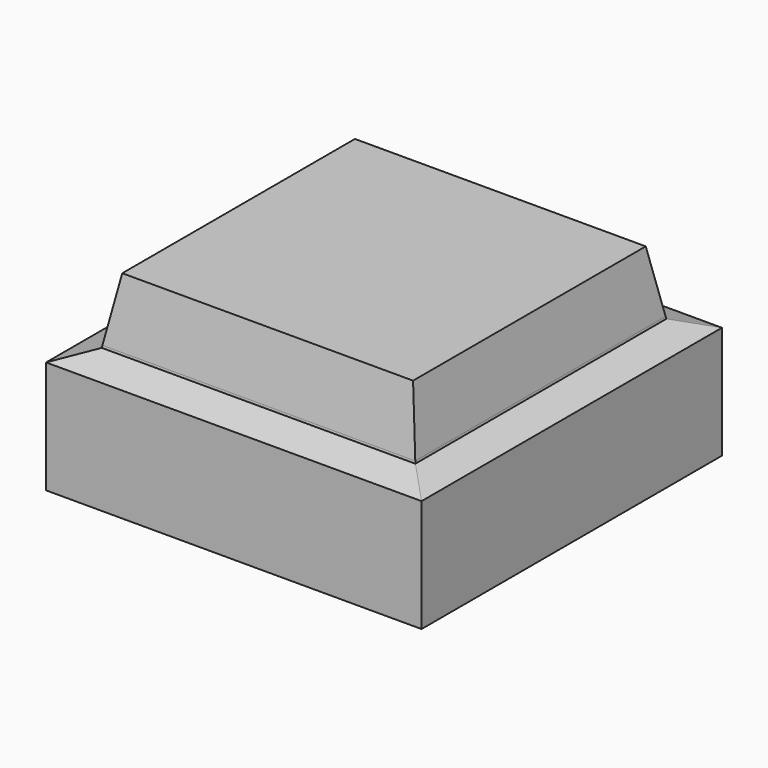
from build123d import *

# Parameters (mm, degrees)
F0_W          = 30
F0_H          = 30
F1_DEPTH      = 10
F2_T          = -2.5
F3_SIZE2      = 7.49999
F3_SIZE       = 0.99999
F4_W          = 25
F4_H          = 25
F5_DEPTH      = 5
F5_TAPER      = 10
F6_T          = 2.5
F6_T3_DEPTH   = 12.6321563139
F6_T5_DEPTH   = 12.6321563139
F6_T7_DEPTH   = 12.6321563139
F6_T9_DEPTH   = 12.6321563139
F6_T11_DEPTH  = 5.00001
F6_T13_DEPTH  = 30
F6_T15_DEPTH  = 30
F7_T4_DEPTH   = 45.5703660639
F7_T10_DEPTH  = 45.5703660639
F7_T16_DEPTH  = 45.5703660639
F7_T23_DEPTH  = 45.5703660639
F7_T29_DEPTH  = 45.5703660639
F7_T35_DEPTH  = 45.5703660639
F7_T41_DEPTH  = 45.5703660639
F7_T47_DEPTH  = 45.5703660639
F7_T54_DEPTH  = 45.5703660639
F7_T60_DEPTH  = 45.5703660639
F7_T66_DEPTH  = 45.5703660639
F7_T72_DEPTH  = 45.5703660639
F7_T78_DEPTH  = 45.5703660639
F7_T85_DEPTH  = 45.5703660639
F7_T91_DEPTH  = 45.5703660639
F7_T97_DEPTH  = 45.5703660639
F7_T103_DEPTH = 45.5703660639
F7_T109_DEPTH = 45.5703660639
F7_T116_DEPTH = 45.5703660639
F7_T122_DEPTH = 45.5703660639
F8_C1_SIZE2   = 1
F8_C1_SIZE    = 1.5
F8_C2_SIZE2   = 1
F8_C2_SIZE    = 1.5
F8_C3_SIZE2   = 1
F8_C3_SIZE    = 1.5
F8_C4_SIZE2   = 1
F8_C4_SIZE    = 1.5


# Not quite as in the source:
# - a fillet or chamfer that OpenCascade refuses, or shapes differently, is made with other operations: its cross-section is extruded or revolved along the edge and cut away or added
# - a fillet or chamfer is up to 0.001 mm smaller than in the source, because OpenCascade refuses the exact size
# - a shell that OpenCascade refuses in one call is made with other operations: the cavity is built on its own and cut out


with BuildPart() as f1:
    # F0 (on Top) → F1 (new body)
    with BuildSketch(Plane.XY):
        with Locations((15, 15)):
            Rectangle(F0_W, F0_H)
    extrude(amount=F1_DEPTH)

    # F2
    f2_openings = [f1.faces().sort_by_distance(p)[0] for p in [
        (15, 15, 0),
    ]]
    offset(amount=F2_T, openings=f2_openings)

    # F3 (size 1 and 7.5 in the source; OpenCascade refuses exactly that, so slightly less here)
    f3_edges = [f1.edges().sort_by_distance(p)[0] for p in [
        (27.5, 15, 0),
        (15, 27.5, 0),
        (2.5, 15, 0),
        (15, 2.5, 0),
    ]]
    chamfer(f3_edges, length=F3_SIZE, length2=F3_SIZE2)

    # F4 (on face) → F5 (join)
    with BuildSketch(Plane.XY.offset(10)):
        with Locations((15, 15)):
            Rectangle(F4_W, F4_H)
    extrude(amount=F5_DEPTH, taper=F5_TAPER)

    # F6: shell of thickness 2.5, made by hand


with BuildPart() as f6_core1:
    # F6_t2: copy of F1
    add(f1.part)

    # the walls: a layer under each face that stays
    f6_faces = [f6_core1.faces().sort_by_distance(p)[0] for p in [
        (1, 1, 0),
        (27.999995, 15, 3.749995),
        (15, 2.000005, 3.749995),
        (15, 27.999995, 3.749995),
        (2.000005, 15, 3.749995),
        (0, 15, 5),
        (15, 0, 5),
        (30, 15, 5),
        (15, 30, 5),
        (27.5, 15, 7.499995),
        (15, 2.5, 7.499995),
        (15, 27.5, 7.499995),
        (2.5, 15, 7.499995),
        (2.1428571429, 2.1428571429, 10),
        (27.0591825482, 15, 12.5),
        (15, 27.0591825482, 12.5),
        (2.9408174518, 15, 12.5),
        (15, 2.9408174518, 12.5),
        (15, 15, 15),
    ]]
    thicken(f6_faces, amount=-F6_T, mode=Mode.SUBTRACT)

    # F6_s4 → F6_t3 (cut)
    with BuildSketch(Plane(origin=(0.7910693611, -0.7910693611, -5.9330716286), x_dir=(-0.7071067812, -0.7071067812, 0), z_dir=(-0.1310232599, 0.1310232599, 0.9826829655))):
        Polygon((-21.2132034356, 18.7255916199), (-22.9654636265, 20.5443932655), (-21.2132034356, 22.2663095063), (-19.4609432447, 20.5443932655), align=None)
    extrude(amount=F6_T3_DEPTH, mode=Mode.SUBTRACT)

    # F6_s6 → F6_t5 (cut)
    with BuildSketch(Plane(origin=(1.3060821999, 1.3060821999, -9.7957013952), x_dir=(0.7071067812, -0.7071067812, 0), z_dir=(-0.1310232599, -0.1310232599, 0.9826829655))):
        Polygon((0, 39.5714452805), (1.7522601909, 41.3902469261), (0, 43.1121631669), (-1.7522601909, 41.3902469261), align=None)
    extrude(amount=F6_T5_DEPTH, mode=Mode.SUBTRACT)

    # F6_s8 → F6_t7 (cut)
    with BuildSketch(Plane(origin=(-0.2760565224, -0.2760565224, -2.0704418621), x_dir=(-0.7071067812, 0.7071067812, 0), z_dir=(0.1310232599, 0.1310232599, 0.9826829655))):
        Polygon((0, -2.1202620407), (-1.7522601909, -0.3014603951), (0, 1.4204558457), (1.7522601909, -0.3014603951), align=None)
    extrude(amount=F6_T7_DEPTH, mode=Mode.SUBTRACT)

    # F6_s10 → F6_t9 (cut)
    with BuildSketch(Plane(origin=(-0.7910693611, 0.7910693611, -5.9330716286), x_dir=(0.7071067812, 0.7071067812, 0), z_dir=(0.1310232599, -0.1310232599, 0.9826829655))):
        Polygon((21.2132034356, 18.7255916199), (22.9654636265, 20.5443932655), (21.2132034356, 22.2663095063), (19.4609432447, 20.5443932655), align=None)
    extrude(amount=F6_T9_DEPTH, mode=Mode.SUBTRACT)

    # F6_s12 → F6_t11 (cut)
    with BuildSketch(Plane.XY.offset(4.99999)):
        Polygon((27.475, 2.525), (30, 2.5), (30, 0), (27.5, 0), align=None)
        Polygon((27.475, 27.475), (30, 27.5), (30, 30), (27.5, 30), align=None)
        Polygon((2.525, 2.525), (2.5, 0), (0, 0), (0, 2.5), align=None)
        Polygon((2.525, 27.475), (2.5, 30), (0, 30), (0, 27.5), align=None)
    extrude(amount=F6_T11_DEPTH, mode=Mode.SUBTRACT)

    # F6_s14 → F6_t13 (cut)
    with BuildSketch(Plane.XZ.offset(-30)):
        Polygon((27.5246201938, 10.0293412044), (27.5, 7.5), (25.4022509221, 7.5), (25.0379806175, 9.5658795558), align=None)
        Polygon((2.4753798062, 10.0293412044), (2.5, 7.5), (4.5977490779, 7.5), (4.9620193825, 9.5658795558), align=None)
    extrude(amount=F6_T13_DEPTH, mode=Mode.SUBTRACT)

    # F6_s16 → F6_t15 (cut)
    with BuildSketch(Plane.YZ):
        Polygon((27.5246201938, 10.0293412044), (27.5, 7.5), (25.4022509221, 7.5), (25.0379806175, 9.5658795558), align=None)
        Polygon((2.4753798062, 10.0293412044), (2.5, 7.5), (4.5977490779, 7.5), (4.9620193825, 9.5658795558), align=None)
    extrude(amount=F6_T15_DEPTH, mode=Mode.SUBTRACT)


with BuildPart() as f1_1:
    add(f1.part)

    # what is left inside the walls is the cavity
    f6_cavity = [f6_core1.part.solids().sort_by_distance(p)[0] for p in [
        (15, 11.532583, 7.525),
    ]]
    add(f6_cavity, mode=Mode.SUBTRACT)

    # F7: chamfer of 1 x 3 on 4 edges, made by hand


with BuildPart() as f7_tool2:
    # F7_s3 → F7_t4 (new body)
    with BuildSketch(Plane.XZ.offset(7.785183032)):
        Polygon((30, 9), (27, 10), (30, 10), align=None)
    extrude(amount=-F7_T4_DEPTH)

    split(bisect_by=Plane(origin=(28.3808742524, 0, 5.0043138668), x_dir=(0, 1, 0), z_dir=(0.984807753, 0, 0.1736481777)), keep=Keep.TOP)

    split(bisect_by=Plane(origin=(0, 0.7145150594, -0.1259882831), x_dir=(1, 0, 0), z_dir=(0, -0.984807753, 0.1736481777)), keep=Keep.TOP)


with BuildPart() as f1_2:
    add(f1_1.part)

    # F7_t1: cut F7_tool2
    add(f7_tool2.part, mode=Mode.SUBTRACT)


with BuildPart() as f7_tool8:
    # F7_s9 → F7_t10 (new body)
    with BuildSketch(Plane.XZ.offset(7.785183032)):
        Polygon((30, 9), (27, 10), (30, 10), align=None)
    extrude(amount=-F7_T10_DEPTH)

    split(bisect_by=Plane(origin=(28.3808742524, 0, 5.0043138668), x_dir=(0, 1, 0), z_dir=(-0.984807753, 0, -0.1736481777)), keep=Keep.TOP)

    split(bisect_by=Plane(origin=(0, 0.7145150594, -0.1259882831), x_dir=(1, 0, 0), z_dir=(0, -0.984807753, 0.1736481777)), keep=Keep.TOP)


with BuildPart() as f1_3:
    add(f1_2.part)

    # F7_t7: cut F7_tool8
    add(f7_tool8.part, mode=Mode.SUBTRACT)


with BuildPart() as f7_tool14:
    # F7_s15 → F7_t16 (new body)
    with BuildSketch(Plane.XZ.offset(7.785183032)):
        Polygon((30, 9), (27, 10), (30, 10), align=None)
    extrude(amount=-F7_T16_DEPTH)

    split(bisect_by=Plane(origin=(28.3808742524, 0, 5.0043138668), x_dir=(0, 1, 0), z_dir=(0.984807753, 0, 0.1736481777)), keep=Keep.TOP)

    split(bisect_by=Plane(origin=(0, 28.3808742524, 5.0043138668), x_dir=(1, 0, 0), z_dir=(0, -0.984807753, -0.1736481777)), keep=Keep.TOP)

    split(bisect_by=Plane(origin=(0, 0.7145150594, -0.1259882831), x_dir=(1, 0, 0), z_dir=(0, 0.984807753, -0.1736481777)), keep=Keep.TOP)


with BuildPart() as f1_4:
    add(f1_3.part)

    # F7_t13: cut F7_tool14
    add(f7_tool14.part, mode=Mode.SUBTRACT)


with BuildPart() as f7_tool21:
    # F7_s22 → F7_t23 (new body)
    with BuildSketch(Plane.XZ.offset(7.785183032)):
        Polygon((30, 9), (27, 10), (30, 10), align=None)
    extrude(amount=-F7_T23_DEPTH)

    split(bisect_by=Plane(origin=(28.3808742524, 0, 5.0043138668), x_dir=(0, 1, 0), z_dir=(0.984807753, 0, 0.1736481777)), keep=Keep.TOP)

    split(bisect_by=Plane(origin=(0, 28.3808742524, 5.0043138668), x_dir=(1, 0, 0), z_dir=(0, 0.984807753, 0.1736481777)), keep=Keep.TOP)


with BuildPart() as f1_5:
    add(f1_4.part)

    # F7_t20: cut F7_tool21
    add(f7_tool21.part, mode=Mode.SUBTRACT)


with BuildPart() as f7_tool27:
    # F7_s28 → F7_t29 (new body)
    with BuildSketch(Plane.XZ.offset(7.785183032)):
        Polygon((30, 9), (27, 10), (30, 10), align=None)
    extrude(amount=-F7_T29_DEPTH)

    split(bisect_by=Plane(origin=(28.3808742524, 0, 5.0043138668), x_dir=(0, 1, 0), z_dir=(-0.984807753, 0, -0.1736481777)), keep=Keep.TOP)

    split(bisect_by=Plane(origin=(0, 28.3808742524, 5.0043138668), x_dir=(1, 0, 0), z_dir=(0, 0.984807753, 0.1736481777)), keep=Keep.TOP)


with BuildPart() as f1_6:
    add(f1_5.part)

    # F7_t26: cut F7_tool27
    add(f7_tool27.part, mode=Mode.SUBTRACT)


with BuildPart() as f7_tool33:
    # F7_s34 → F7_t35 (new body)
    with BuildSketch(Plane.YZ.offset(-7.785183032)):
        Polygon((0, 9), (3, 10), (0, 10), align=None)
    extrude(amount=F7_T35_DEPTH)

    split(bisect_by=Plane(origin=(0.7145150594, 0, -0.1259882831), x_dir=(0, 1, 0), z_dir=(-0.984807753, 0, 0.1736481777)), keep=Keep.TOP)

    split(bisect_by=Plane(origin=(0, 0.7145150594, -0.1259882831), x_dir=(1, 0, 0), z_dir=(0, -0.984807753, 0.1736481777)), keep=Keep.TOP)


with BuildPart() as f1_7:
    add(f1_6.part)

    # F7_t32: cut F7_tool33
    add(f7_tool33.part, mode=Mode.SUBTRACT)


with BuildPart() as f7_tool39:
    # F7_s40 → F7_t41 (new body)
    with BuildSketch(Plane.YZ.offset(-7.785183032)):
        Polygon((0, 9), (3, 10), (0, 10), align=None)
    extrude(amount=F7_T41_DEPTH)

    split(bisect_by=Plane(origin=(0.7145150594, 0, -0.1259882831), x_dir=(0, 1, 0), z_dir=(-0.984807753, 0, 0.1736481777)), keep=Keep.TOP)

    split(bisect_by=Plane(origin=(0, 0.7145150594, -0.1259882831), x_dir=(1, 0, 0), z_dir=(0, 0.984807753, -0.1736481777)), keep=Keep.TOP)


with BuildPart() as f1_8:
    add(f1_7.part)

    # F7_t38: cut F7_tool39
    add(f7_tool39.part, mode=Mode.SUBTRACT)


with BuildPart() as f7_tool45:
    # F7_s46 → F7_t47 (new body)
    with BuildSketch(Plane.YZ.offset(-7.785183032)):
        Polygon((0, 9), (3, 10), (0, 10), align=None)
    extrude(amount=F7_T47_DEPTH)

    split(bisect_by=Plane(origin=(28.3808742524, 0, 5.0043138668), x_dir=(0, 1, 0), z_dir=(-0.984807753, 0, -0.1736481777)), keep=Keep.TOP)

    split(bisect_by=Plane(origin=(0.7145150594, 0, -0.1259882831), x_dir=(0, 1, 0), z_dir=(0.984807753, 0, -0.1736481777)), keep=Keep.TOP)

    split(bisect_by=Plane(origin=(0, 0.7145150594, -0.1259882831), x_dir=(1, 0, 0), z_dir=(0, -0.984807753, 0.1736481777)), keep=Keep.TOP)


with BuildPart() as f1_9:
    add(f1_8.part)

    # F7_t44: cut F7_tool45
    add(f7_tool45.part, mode=Mode.SUBTRACT)


with BuildPart() as f7_tool52:
    # F7_s53 → F7_t54 (new body)
    with BuildSketch(Plane.YZ.offset(-7.785183032)):
        Polygon((0, 9), (3, 10), (0, 10), align=None)
    extrude(amount=F7_T54_DEPTH)

    split(bisect_by=Plane(origin=(28.3808742524, 0, 5.0043138668), x_dir=(0, 1, 0), z_dir=(0.984807753, 0, 0.1736481777)), keep=Keep.TOP)

    split(bisect_by=Plane(origin=(0, 0.7145150594, -0.1259882831), x_dir=(1, 0, 0), z_dir=(0, -0.984807753, 0.1736481777)), keep=Keep.TOP)


with BuildPart() as f1_10:
    add(f1_9.part)

    # F7_t51: cut F7_tool52
    add(f7_tool52.part, mode=Mode.SUBTRACT)


with BuildPart() as f7_tool58:
    # F7_s59 → F7_t60 (new body)
    with BuildSketch(Plane.YZ.offset(-7.785183032)):
        Polygon((0, 9), (3, 10), (0, 10), align=None)
    extrude(amount=F7_T60_DEPTH)

    split(bisect_by=Plane(origin=(28.3808742524, 0, 5.0043138668), x_dir=(0, 1, 0), z_dir=(0.984807753, 0, 0.1736481777)), keep=Keep.TOP)

    split(bisect_by=Plane(origin=(0, 0.7145150594, -0.1259882831), x_dir=(1, 0, 0), z_dir=(0, 0.984807753, -0.1736481777)), keep=Keep.TOP)


with BuildPart() as f1_11:
    add(f1_10.part)

    # F7_t57: cut F7_tool58
    add(f7_tool58.part, mode=Mode.SUBTRACT)


with BuildPart() as f7_tool64:
    # F7_s65 → F7_t66 (new body)
    with BuildSketch(Plane.XZ.offset(-37.785183032)):
        Polygon((0, 9), (3, 10), (0, 10), align=None)
    extrude(amount=F7_T66_DEPTH)

    split(bisect_by=Plane(origin=(0, 28.3808742524, 5.0043138668), x_dir=(1, 0, 0), z_dir=(0, 0.984807753, 0.1736481777)), keep=Keep.TOP)

    split(bisect_by=Plane(origin=(0.7145150594, 0, -0.1259882831), x_dir=(0, 1, 0), z_dir=(-0.984807753, 0, 0.1736481777)), keep=Keep.TOP)


with BuildPart() as f1_12:
    add(f1_11.part)

    # F7_t63: cut F7_tool64
    add(f7_tool64.part, mode=Mode.SUBTRACT)


with BuildPart() as f7_tool70:
    # F7_s71 → F7_t72 (new body)
    with BuildSketch(Plane.XZ.offset(-37.785183032)):
        Polygon((0, 9), (3, 10), (0, 10), align=None)
    extrude(amount=F7_T72_DEPTH)

    split(bisect_by=Plane(origin=(0, 28.3808742524, 5.0043138668), x_dir=(1, 0, 0), z_dir=(0, 0.984807753, 0.1736481777)), keep=Keep.TOP)

    split(bisect_by=Plane(origin=(0.7145150594, 0, -0.1259882831), x_dir=(0, 1, 0), z_dir=(0.984807753, 0, -0.1736481777)), keep=Keep.TOP)


with BuildPart() as f1_13:
    add(f1_12.part)

    # F7_t69: cut F7_tool70
    add(f7_tool70.part, mode=Mode.SUBTRACT)


with BuildPart() as f7_tool76:
    # F7_s77 → F7_t78 (new body)
    with BuildSketch(Plane.XZ.offset(-37.785183032)):
        Polygon((0, 9), (3, 10), (0, 10), align=None)
    extrude(amount=F7_T78_DEPTH)

    split(bisect_by=Plane(origin=(0, 28.3808742524, 5.0043138668), x_dir=(1, 0, 0), z_dir=(0, -0.984807753, -0.1736481777)), keep=Keep.TOP)

    split(bisect_by=Plane(origin=(0.7145150594, 0, -0.1259882831), x_dir=(0, 1, 0), z_dir=(-0.984807753, 0, 0.1736481777)), keep=Keep.TOP)

    split(bisect_by=Plane(origin=(0, 0.7145150594, -0.1259882831), x_dir=(1, 0, 0), z_dir=(0, 0.984807753, -0.1736481777)), keep=Keep.TOP)


with BuildPart() as f1_14:
    add(f1_13.part)

    # F7_t75: cut F7_tool76
    add(f7_tool76.part, mode=Mode.SUBTRACT)


with BuildPart() as f7_tool83:
    # F7_s84 → F7_t85 (new body)
    with BuildSketch(Plane.XZ.offset(-37.785183032)):
        Polygon((0, 9), (3, 10), (0, 10), align=None)
    extrude(amount=F7_T85_DEPTH)

    split(bisect_by=Plane(origin=(0.7145150594, 0, -0.1259882831), x_dir=(0, 1, 0), z_dir=(-0.984807753, 0, 0.1736481777)), keep=Keep.TOP)

    split(bisect_by=Plane(origin=(0, 0.7145150594, -0.1259882831), x_dir=(1, 0, 0), z_dir=(0, -0.984807753, 0.1736481777)), keep=Keep.TOP)


with BuildPart() as f1_15:
    add(f1_14.part)

    # F7_t82: cut F7_tool83
    add(f7_tool83.part, mode=Mode.SUBTRACT)


with BuildPart() as f7_tool89:
    # F7_s90 → F7_t91 (new body)
    with BuildSketch(Plane.XZ.offset(-37.785183032)):
        Polygon((0, 9), (3, 10), (0, 10), align=None)
    extrude(amount=F7_T91_DEPTH)

    split(bisect_by=Plane(origin=(0.7145150594, 0, -0.1259882831), x_dir=(0, 1, 0), z_dir=(0.984807753, 0, -0.1736481777)), keep=Keep.TOP)

    split(bisect_by=Plane(origin=(0, 0.7145150594, -0.1259882831), x_dir=(1, 0, 0), z_dir=(0, -0.984807753, 0.1736481777)), keep=Keep.TOP)


with BuildPart() as f1_16:
    add(f1_15.part)

    # F7_t88: cut F7_tool89
    add(f7_tool89.part, mode=Mode.SUBTRACT)


with BuildPart() as f7_tool95:
    # F7_s96 → F7_t97 (new body)
    with BuildSketch(Plane.YZ.offset(37.785183032)):
        Polygon((30, 9), (27, 10), (30, 10), align=None)
    extrude(amount=-F7_T97_DEPTH)

    split(bisect_by=Plane(origin=(28.3808742524, 0, 5.0043138668), x_dir=(0, 1, 0), z_dir=(0.984807753, 0, 0.1736481777)), keep=Keep.TOP)

    split(bisect_by=Plane(origin=(0, 28.3808742524, 5.0043138668), x_dir=(1, 0, 0), z_dir=(0, 0.984807753, 0.1736481777)), keep=Keep.TOP)


with BuildPart() as f1_17:
    add(f1_16.part)

    # F7_t94: cut F7_tool95
    add(f7_tool95.part, mode=Mode.SUBTRACT)


with BuildPart() as f7_tool101:
    # F7_s102 → F7_t103 (new body)
    with BuildSketch(Plane.YZ.offset(37.785183032)):
        Polygon((30, 9), (27, 10), (30, 10), align=None)
    extrude(amount=-F7_T103_DEPTH)

    split(bisect_by=Plane(origin=(28.3808742524, 0, 5.0043138668), x_dir=(0, 1, 0), z_dir=(0.984807753, 0, 0.1736481777)), keep=Keep.TOP)

    split(bisect_by=Plane(origin=(0, 28.3808742524, 5.0043138668), x_dir=(1, 0, 0), z_dir=(0, -0.984807753, -0.1736481777)), keep=Keep.TOP)


with BuildPart() as f1_18:
    add(f1_17.part)

    # F7_t100: cut F7_tool101
    add(f7_tool101.part, mode=Mode.SUBTRACT)


with BuildPart() as f7_tool107:
    # F7_s108 → F7_t109 (new body)
    with BuildSketch(Plane.YZ.offset(37.785183032)):
        Polygon((30, 9), (27, 10), (30, 10), align=None)
    extrude(amount=-F7_T109_DEPTH)

    split(bisect_by=Plane(origin=(28.3808742524, 0, 5.0043138668), x_dir=(0, 1, 0), z_dir=(-0.984807753, 0, -0.1736481777)), keep=Keep.TOP)

    split(bisect_by=Plane(origin=(0, 28.3808742524, 5.0043138668), x_dir=(1, 0, 0), z_dir=(0, 0.984807753, 0.1736481777)), keep=Keep.TOP)

    split(bisect_by=Plane(origin=(0.7145150594, 0, -0.1259882831), x_dir=(0, 1, 0), z_dir=(0.984807753, 0, -0.1736481777)), keep=Keep.TOP)


with BuildPart() as f1_19:
    add(f1_18.part)

    # F7_t106: cut F7_tool107
    add(f7_tool107.part, mode=Mode.SUBTRACT)


with BuildPart() as f7_tool114:
    # F7_s115 → F7_t116 (new body)
    with BuildSketch(Plane.YZ.offset(37.785183032)):
        Polygon((30, 9), (27, 10), (30, 10), align=None)
    extrude(amount=-F7_T116_DEPTH)

    split(bisect_by=Plane(origin=(0, 28.3808742524, 5.0043138668), x_dir=(1, 0, 0), z_dir=(0, 0.984807753, 0.1736481777)), keep=Keep.TOP)

    split(bisect_by=Plane(origin=(0.7145150594, 0, -0.1259882831), x_dir=(0, 1, 0), z_dir=(-0.984807753, 0, 0.1736481777)), keep=Keep.TOP)


with BuildPart() as f1_20:
    add(f1_19.part)

    # F7_t113: cut F7_tool114
    add(f7_tool114.part, mode=Mode.SUBTRACT)


with BuildPart() as f7_tool120:
    # F7_s121 → F7_t122 (new body)
    with BuildSketch(Plane.YZ.offset(37.785183032)):
        Polygon((30, 9), (27, 10), (30, 10), align=None)
    extrude(amount=-F7_T122_DEPTH)

    split(bisect_by=Plane(origin=(0, 28.3808742524, 5.0043138668), x_dir=(1, 0, 0), z_dir=(0, -0.984807753, -0.1736481777)), keep=Keep.TOP)

    split(bisect_by=Plane(origin=(0.7145150594, 0, -0.1259882831), x_dir=(0, 1, 0), z_dir=(-0.984807753, 0, 0.1736481777)), keep=Keep.TOP)


with BuildPart() as f1_21:
    add(f1_20.part)

    # F7_t119: cut F7_tool120
    add(f7_tool120.part, mode=Mode.SUBTRACT)

    # F8: chamfer of 1 x 1.5 on 4 edges, made by hand

    # F8_c1
    f8_c1_edges = [f1_21.edges().sort_by_distance(p)[0] for p in [
        (28.49999, 15, 0),
    ]]
    f8_c1_side = f1_21.faces().sort_by_distance((28.51999, 15, 0))[0]
    chamfer(f8_c1_edges, length=F8_C1_SIZE, length2=F8_C1_SIZE2, reference=f8_c1_side)

    # F8_c2
    f8_c2_edges = [f1_21.edges().sort_by_distance(p)[0] for p in [
        (15, 1.50001, 0),
    ]]
    f8_c2_side = f1_21.faces().sort_by_distance((15, 1.48001, 0))[0]
    chamfer(f8_c2_edges, length=F8_C2_SIZE, length2=F8_C2_SIZE2, reference=f8_c2_side)

    # F8_c3
    f8_c3_edges = [f1_21.edges().sort_by_distance(p)[0] for p in [
        (15, 28.49999, 0),
    ]]
    f8_c3_side = f1_21.faces().sort_by_distance((15, 28.51999, 0))[0]
    chamfer(f8_c3_edges, length=F8_C3_SIZE, length2=F8_C3_SIZE2, reference=f8_c3_side)

    # F8_c4
    f8_c4_edges = [f1_21.edges().sort_by_distance(p)[0] for p in [
        (1.50001, 15, 0),
    ]]
    f8_c4_side = f1_21.faces().sort_by_distance((1.48001, 15, 0))[0]
    chamfer(f8_c4_edges, length=F8_C4_SIZE, length2=F8_C4_SIZE2, reference=f8_c4_side)


solid = f1_21.part
